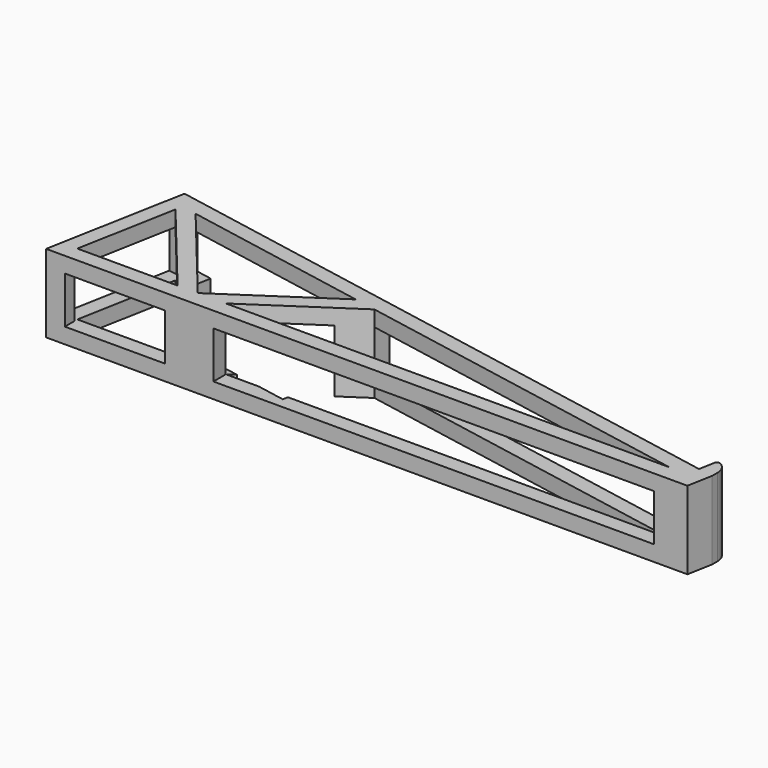
from build123d import *

# Parameters (mm, degrees)
F1_DEPTH     = 25
F3_W         = 103.0636096465
F3_H         = 15
F3_W_2       = 5
F3_W_3       = 5.0301977637
F4_DEPTH     = 29.1
F5_W         = 32.1414392277
F5_H         = 15
F5_W_2       = 37.424231063
F6_DEPTH     = 5
F8_W         = 35.7737973711
F8_H         = 15
F9_DEPTH     = 25
F10_T1_DEPTH = 45.720844557
F11_R        = 1
F12_W        = 15.2368300635
F12_H        = 15
F13_DEPTH    = 30


# Not quite as in the source:
# - a fillet or chamfer that OpenCascade refuses, or shapes differently, is made with other operations: its cross-section is extruded or revolved along the edge and cut away or added


with BuildPart() as f1:
    # F0 (on Top) → F1 (new body)
    with BuildSketch(Plane.XY):
        Polygon((-57.4114776212, 45), (-65.7924397243, 0), (139.809737024, 0), (141.2981229206, 7.9916081853), (136.3826469731, 8.9070841327), align=None)
        Polygon((18.9005100522, 25.701403032), (130.0528008015, 5), (-12.1503930873, 5), (-21.1640298367, 5), (-27.6338049994, 5), (-59.7752442271, 5), (-53.8331571099, 36.9049193859), (-53.4114776212, 39.1690481052), (-48.4663143975, 38.2480430925), (11.8550538619, 27.0135741727), align=None, mode=Mode.SUBTRACT)
        Polygon((136.3826469731, 8.9070841327), (141.2981229206, 7.9916081853), (141.2981229206, 14.3588015401), (137.528741777, 15.0608246626), align=None)
        Polygon((-27.6338049994, 5), (-21.1640298367, 5), (-48.4663143975, 38.2480430925), (-53.4114776212, 39.1690481052), (-53.8331571099, 36.9049193859), align=None)
        Polygon((-12.1503930873, 5), (18.9005100522, 25.701403032), (11.8550538619, 27.0135741727), (-21.1640298367, 5), align=None)
    extrude(amount=F1_DEPTH)

    # F3 (on offset) → F4 (cut)
    with BuildSketch(Plane(origin=(6.1753463271, 33.1573608496, 0), x_dir=(-0.9830951895, 0.1830951895, 0), z_dir=(0.1830951895, 0.9830951895, 0))):
        with Locations((-70.4070020763, 12.5)):
            Rectangle(F3_W, F3_H)
        Polygon((49.6500332337, 20), (-1.7085909409, 20), (-1.7085909409, 5), (0, 5), (49.6500332337, 5), align=None)
        with Locations((-124.4388068995, 12.5)):
            Rectangle(F3_W_2, F3_H)
        with Locations((-16.375197253, 12.5)):
            Rectangle(F3_W_2, F3_H)
        Polygon((-1.7085909409, 20), (-6.7085909409, 20), (-6.7085909409, 0), (54.6500332337, 0), (54.6500332337, 5), (49.6500332337, 5), (0, 5), (-1.7085909409, 5), align=None)
        with Locations((52.1500332337, 12.5)):
            Rectangle(F3_W_2, F3_H)
        with Locations((57.1651321155, 12.5)):
            Rectangle(F3_W_3, F3_H)
    extrude(amount=-F4_DEPTH, mode=Mode.SUBTRACT)

    # F5 (on Front) → F6 (cut)
    with BuildSketch(Plane.XZ):
        with Locations((-43.7045246133, 12.5)):
            Rectangle(F5_W, F5_H)
        with Locations((6.5617224442, 12.5)):
            Rectangle(F5_W_2, F5_H)
    extrude(amount=-F6_DEPTH, mode=Mode.SUBTRACT)

    # F8 (on offset) → F9 (cut)
    with BuildSketch(Plane(origin=(-63.5868239483, 11.8426391504, 0), x_dir=(-0.1830951895, -0.9830951895, 0), z_dir=(-0.9830951895, 0.1830951895, 0))):
        with Locations((-10.8406194676, 12.5)):
            Rectangle(F8_W, F8_H)
    extrude(amount=-F9_DEPTH, mode=Mode.SUBTRACT)

    # F10: fillet of radius 5 on 1 edges, made by hand

    # F10_s2 → F10_t1 (cut)
    with BuildSketch(Plane.XY.offset(-10.3604222785)):
        with BuildLine():
            ThreePointArc((141.2981229206, 10.2146326287), (140.2448363813, 13.2843969289), (137.528741777, 15.0608246626))
            Line((137.528741777, 15.0608246626), (141.2981229206, 14.3588015401))
            Line((141.2981229206, 14.3588015401), (141.2981229206, 10.2146326287))
        make_face()
    extrude(amount=F10_T1_DEPTH, mode=Mode.SUBTRACT)

    # F11
    f11_edges = [f1.edges().sort_by_distance(p)[0] for p in [
        (137.528742, 15.060825, 12.5),
    ]]
    fillet(f11_edges, radius=F11_R)

    # F12 (on Right) → F13 (cut)
    with BuildSketch(Plane.YZ):
        with Locations((12.5338909792, 12.5)):
            Rectangle(F12_W, F12_H)
    extrude(amount=-F13_DEPTH, mode=Mode.SUBTRACT)


solid = f1.part
